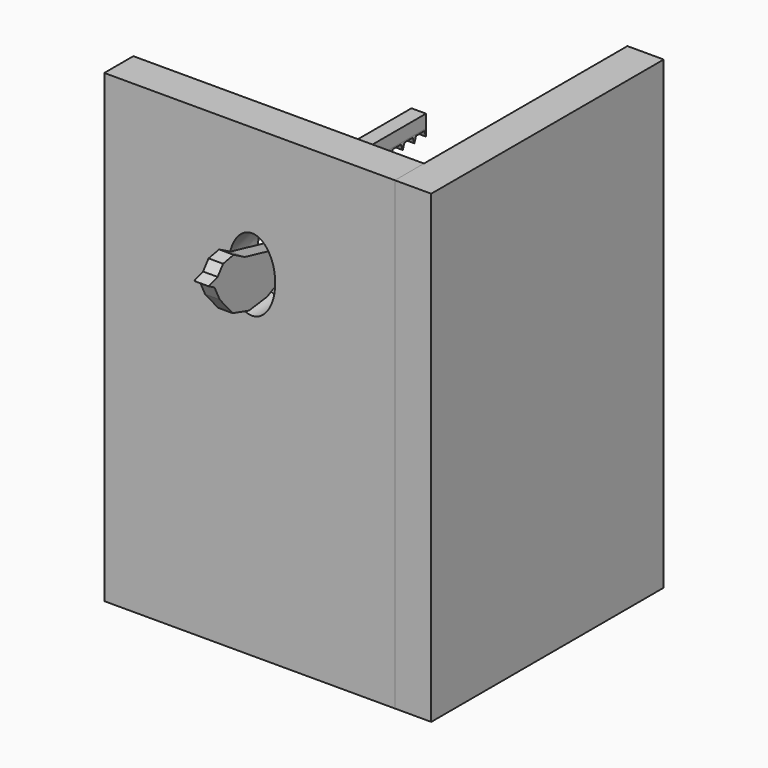
from build123d import *

# Parameters (mm, degrees)
F2_DEPTH      = 3.175
F2_DEPTH_BACK = 3.175
F3_W          = 127
F3_H          = 203.2
F4_DEPTH      = 15.875
F5_W          = 127
F5_H          = 203.2
F6_DEPTH      = 15.875
F7_W          = 1.9345794022
F7_H          = 2.1087378263
F8_DEPTH      = 5.1
F8_DEPTH_BACK = 5.1
F10_DEPTH     = 6.35


# Not quite as in the source:
# - a variable given as a bare number and used for a length is read in inches; the dataset says mm whatever the document's units were


with BuildPart() as f2:
    # F1 (on Right) → F2 (new body, two sides)
    with BuildSketch(Plane.YZ) as f2_sk:
        Polygon((-38.594293431, 41.0619944761), (-43.4932071195, 39.4476822198), (-40.3047855642, 37.7265355505), (-37.482474095, 31.9108637659), (-30.3839322929, 23.7697052669), (-21.4893757698, 21.1347664927), (-11.6540487569, 22.4176353632), (-3.8713104227, 26.0096677876), (1.5612775253, 30.1139711279), (3.4430737253, 30.3825888026), (19.4908740901, 30.3825888026), (19.4908740901, 9.2737668518), (75.5363102326, 9.2737668518), (75.5363102326, 15.1181869977), (22.9848847986, 15.1181869977), (22.9848847986, 30.3825888026), (23.0121565767, 36.6700449444), (23.0121565767, 51.9156488357), (75.233297396, 51.9156488357), (75.233297396, 57.6085964854), (19.9154892202, 57.6085964854), (19.9154892202, 36.6700449444), (1.8303633194, 36.6700449444), (-23.7130144418, 42.6869621861), (-29.8707857541, 46.0224201941), (-35.6009331156, 44.9106008581), align=None)
    extrude(amount=F2_DEPTH)
    extrude(f2_sk.sketch, amount=-F2_DEPTH_BACK)


with BuildPart() as f4:
    # F3 (on Front) → F4 (new body)
    with BuildSketch(Plane.XZ):
        with Locations((-1.0310392827, -13.3170386252)):
            Rectangle(F3_W, F3_H)
        with BuildLine():
            add(Edge.make_bspline(
                [(0, 15.875), (17.626948032, 15.875), (8.813474016, 39.6875), (0, 63.5), (-8.813474016, 39.6875), (-17.626948032, 15.875), (0, 15.875)],
                knots=[0, 0, 0, 2.0943951024, 2.0943951024, 4.1887902048, 4.1887902048, 6.2831853072, 6.2831853072, 6.2831853072], degree=2, weights=[1, 0.5, 1, 0.5, 1, 0.5, 1]))
        make_face(mode=Mode.SUBTRACT)
    extrude(amount=F4_DEPTH)


with BuildPart() as f6:
    # F5 (on face) → F6 (new body)
    with BuildSketch(Plane.YZ.offset(62.4689607173)):
        with Locations((47.625, -13.3170386252)):
            Rectangle(F5_W, F5_H)
    extrude(amount=F6_DEPTH)


with BuildPart() as f8:
    # F7 (on Right) → F8 (new body, two sides)
    with BuildSketch(Plane.YZ) as f8_sk:
        Polygon((16, 56.2037155032), (16, 77.0455870458), (0, 77.0455870458), (0, 49.0455870458), (16, 49.0455870458), (16, 54.0949776769), align=None)
        with Locations((16.9672897011, 55.14934659)):
            Rectangle(F7_W, F7_H)
    extrude(amount=F8_DEPTH)
    extrude(f8_sk.sketch, amount=-F8_DEPTH_BACK)


with BuildPart() as f10:
    # F9 (on face) → F10 (new body)
    with BuildSketch(Plane(origin=(-3.175, 0, 0), x_dir=(0, -1, 0), z_dir=(-1, 0, 0))):
        Polygon((-68.883297396, 51.9156488357), (-75.233297396, 51.9156488357), (-75.233297396, 51.2806488357), (-75.233297396, 48.7406488357), (-74.308813001, 51.2806488357), (-69.807781791, 51.2806488357), (-68.883297396, 48.7406488357), (-68.883297396, 51.2806488357), align=None)
        Polygon((-62.533297396, 51.9156488357), (-68.883297396, 51.9156488357), (-68.883297396, 51.2806488357), (-68.883297396, 48.7406488357), (-67.958813001, 51.2806488357), (-63.457781791, 51.2806488357), (-62.533297396, 48.7406488357), (-62.533297396, 51.2806488357), align=None)
        Polygon((-56.183297396, 51.9156488357), (-62.533297396, 51.9156488357), (-62.533297396, 51.2806488357), (-62.533297396, 48.7406488357), (-61.608813001, 51.2806488357), (-57.107781791, 51.2806488357), (-56.183297396, 48.7406488357), (-56.183297396, 51.2806488357), align=None)
        Polygon((-49.833297396, 51.9156488357), (-56.183297396, 51.9156488357), (-56.183297396, 51.2806488357), (-56.183297396, 48.7406488357), (-55.258813001, 51.2806488357), (-50.757781791, 51.2806488357), (-49.833297396, 48.7406488357), (-49.833297396, 51.2806488357), align=None)
        Polygon((-43.483297396, 51.9156488357), (-49.833297396, 51.9156488357), (-49.833297396, 51.2806488357), (-49.833297396, 48.7406488357), (-48.908813001, 51.2806488357), (-44.407781791, 51.2806488357), (-43.483297396, 48.7406488357), (-43.483297396, 51.2806488357), align=None)
        Polygon((-37.133297396, 51.9156488357), (-43.483297396, 51.9156488357), (-43.483297396, 51.2806488357), (-43.483297396, 48.7406488357), (-42.558813001, 51.2806488357), (-38.057781791, 51.2806488357), (-37.133297396, 48.7406488357), (-37.133297396, 51.2806488357), align=None)
        Polygon((-30.783297396, 51.9156488357), (-37.133297396, 51.9156488357), (-37.133297396, 51.2806488357), (-37.133297396, 48.7406488357), (-36.208813001, 51.2806488357), (-31.707781791, 51.2806488357), (-30.783297396, 48.7406488357), (-30.783297396, 51.2806488357), align=None)
        Polygon((-24.433297396, 51.9156488357), (-30.783297396, 51.9156488357), (-30.783297396, 51.2806488357), (-30.783297396, 48.7406488357), (-29.858813001, 51.2806488357), (-25.357781791, 51.2806488357), (-24.433297396, 48.7406488357), (-24.433297396, 51.2806488357), align=None)
    extrude(amount=-F10_DEPTH)


solid = Compound([f2.part, f4.part, f6.part, f8.part, f10.part])
